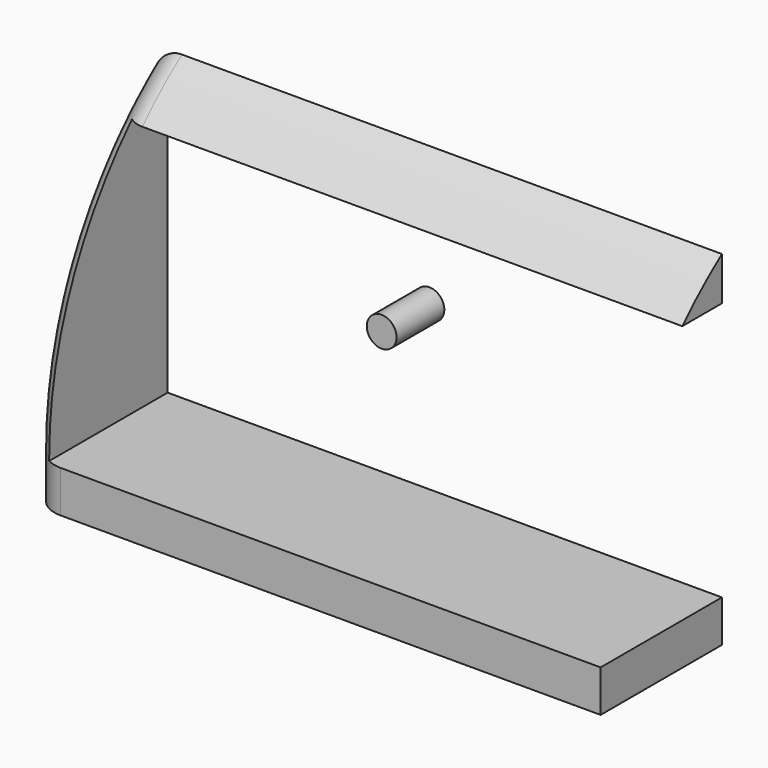
from build123d import *

# Parameters (mm, degrees)
F0_R        = 2.5
F1_DEPTH    = 10
F3_DEPTH    = 25.4
F4_T1_DEPTH = 345.5970234227
F5_T1_DEPTH = 20.3399448702
F5_T4_ANGLE = 65.6015156343


# Not quite as in the source:
# - a fillet or chamfer that OpenCascade refuses, or shapes differently, is made with other operations: its cross-section is extruded or revolved along the edge and cut away or added


with BuildPart() as f1:
    # F0 (on Front) → F1 (new body)
    with BuildSketch(Plane.XZ):
        Circle(F0_R)
    extrude(amount=F1_DEPTH)


with BuildPart() as f3:
    # F2 (on Front) → F3 (new body)
    with BuildSketch(Plane.XZ):
        Polygon((-43.8486076891, -27.3053273559), (-43.8486076891, 16.0576831549), (49.0021444857, 16.0576831549), (49.0021444857, 23.334402591), (-46.5399287641, 23.334402591), (-46.5399287641, -34.3165323138), (49.0021444857, -34.3165323138), (49.0021444857, -27.3053273559), align=None)
    extrude(amount=F3_DEPTH)

    # F4: fillet of radius 61.9342347291 on 1 edges, made by hand

    # F4_s2 → F4_t1 (cut)
    with BuildSketch(Plane.YZ.offset(-171.5674038506)):
        with BuildLine():
            ThreePointArc((0, 23.334402591), (-18.6860935062, 1.369174822), (-25.4, -26.6765874436))
            Line((-25.4, -26.6765874436), (-25.4, 23.334402591))
            Line((-25.4, 23.334402591), (0, 23.334402591))
        make_face()
    extrude(amount=F4_T1_DEPTH, mode=Mode.SUBTRACT)

    # F5: fillet of radius 5.08 on 2 edges, made by hand

    # F5_s2 → F5_t1 (cut)
    with BuildSketch(Plane.XY.offset(-47.0165323138)):
        with BuildLine():
            ThreePointArc((-41.4599287641, -25.4), (-45.0520312125, -23.9121024484), (-46.5399287641, -20.32))
            Line((-46.5399287641, -20.32), (-46.5399287641, -25.4))
            Line((-46.5399287641, -25.4), (-41.4599287641, -25.4))
        make_face()
    extrude(amount=F5_T1_DEPTH, mode=Mode.SUBTRACT)

    # F5_s3 → F5_t4 (revolve, cut)
    with BuildSketch(Plane.XY.offset(-26.6765874438)):
        with BuildLine():
            ThreePointArc((-41.4599287641, -25.4), (-45.0520312125, -23.9121024484), (-46.5399287641, -20.32))
            Line((-46.5399287641, -20.32), (-46.5399287641, -25.4))
            Line((-46.5399287641, -25.4), (-41.4599287641, -25.4))
        make_face()
    revolve(axis=Axis((-46.5399287641, 36.5342347296, -26.6765874438), (-1, 0, 0)), revolution_arc=F5_T4_ANGLE, mode=Mode.SUBTRACT)


solid = Compound([f1.part, f3.part])
